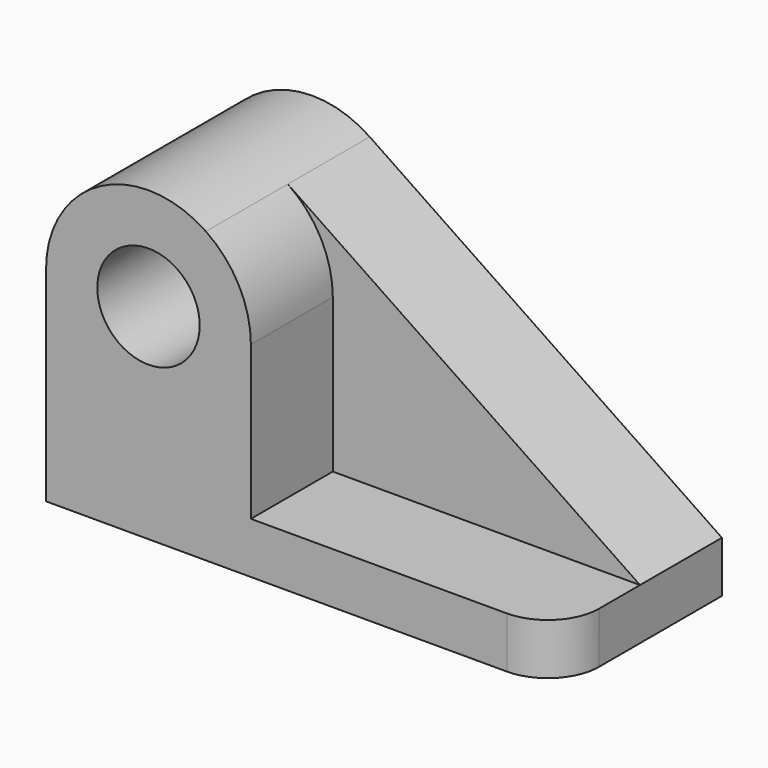
from build123d import *
from build123d import SkipClean  # not in build123d's __all__

# Parameters (mm, degrees)
F1_DEPTH = 25.4
F2_R     = 12.7
F3_DEPTH = 25.4
F4_R     = 12.7


with BuildPart() as f1:
    # F0 (on Front) → F1 (new body)
    with BuildSketch(Plane.XZ):
        with BuildLine():
            ThreePointArc((-43.6412656098, 69.364863438), (-69.7853980696, 70.7671344092), (-83.2791387379, 48.3305350963))
            Line((-83.2791387379, 48.3305350963), (-83.2791387379, -2.4694649037))
            Line((-83.2791387379, -2.4694649037), (43.7208612621, -2.4694649037))
            Line((43.7208612621, -2.4694649037), (43.7208612621, 10.2305350963))
            Line((43.7208612621, 10.2305350963), (-43.6412656098, 69.364863438))
        make_face()
        with BuildLine():
            ThreePointArc((-70.5791387379, 48.3305350963), (-57.8791387379, 61.0305350963), (-45.1791387379, 48.3305350963))
            ThreePointArc((-45.1791387379, 48.3305350963), (-57.8791387379, 35.6305350963), (-70.5791387379, 48.3305350963))
        make_face(mode=Mode.SUBTRACT)
    extrude(amount=F1_DEPTH)

    # F2 (on face) → F3 (join)
    with BuildSketch(Plane.XZ.offset(25.4)):
        with BuildLine():
            Line((-32.4791387379, 10.2305350963), (-32.4791387379, 48.3305350963))
            ThreePointArc((-32.4791387379, 48.3305350963), (-35.442539425, 60.236794428), (-43.6412656098, 69.364863438))
            ThreePointArc((-43.6412656098, 69.364863438), (-69.7853980696, 70.7671344092), (-83.2791387379, 48.3305350963))
            Line((-83.2791387379, 48.3305350963), (-83.2791387379, 10.2305350963))
            Line((-83.2791387379, 10.2305350963), (-83.2791387379, -2.4694649037))
            Line((-83.2791387379, -2.4694649037), (43.7208612621, -2.4694649037))
            Line((43.7208612621, -2.4694649037), (43.7208612621, 10.2305350963))
            Line((43.7208612621, 10.2305350963), (-32.4791387379, 10.2305350963))
        make_face()
        with Locations((-57.8791387379, 48.3305350963)):
            Circle(F2_R, mode=Mode.SUBTRACT)
    with SkipClean():  # cleaning this boolean's faces spoils the solid; the shape is the same uncleaned
        extrude(amount=F3_DEPTH)

    # F4
    f4_edges = [f1.edges().sort_by_distance(p)[0] for p in [
        (43.720861, -50.8, 3.880535),
    ]]
    fillet(f4_edges, radius=F4_R)


solid = f1.part
